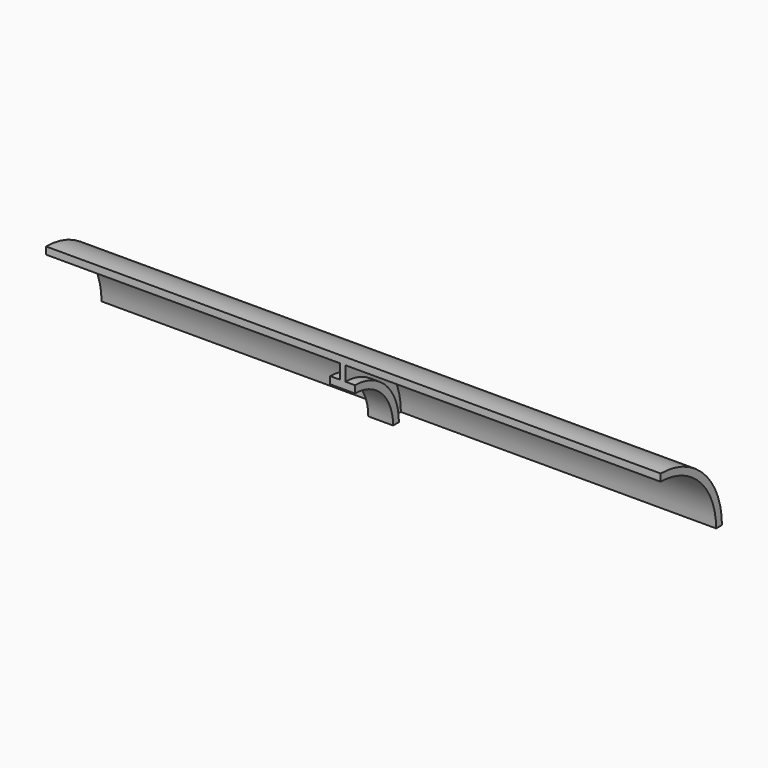
from build123d import *

# Parameters (mm, degrees)
F4_DEPTH = 1877.2339820862
F5_DEPTH = 1745.1422214508


# Not quite as in the source:
# - a feature of the source that left no trace in its solid (it failed there, or was rolled back) is left out


with BuildPart() as f2:
    # F2: sweep along a path in F1
    with BuildLine(Plane.YZ) as f2_path:
        ThreePointArc((0, 0), (269.4076836321, -111.5923163679), (381, -381))
    # F0 (on Front) → F2 (sweep)
    with BuildSketch(Plane.XZ):
        Polygon((76.2, 88.9), (0, 88.9), (-76.2, 88.9), (-76.2, 44.45), (-17.3748321831, 44.45), (-17.3748321831, 0), (-17.3748321831, -44.45), (-76.2, -44.45), (-76.2, -88.9), (0, -88.9), (76.2, -88.9), (76.2, -44.45), (17.3748321831, -44.45), (17.3748321831, 0), (17.3748321831, 44.45), (76.2, 44.45), align=None)
    sweep(path=f2_path.line)

    # F4 (add): a face of the model
    f4_faces = [f2.faces().sort_by_distance(p)[0] for p in [
        (76.2, 305.5375800558, -75.4624199442),
    ]]
    extrude(f4_faces, amount=F4_DEPTH)

    # F3 (on face) → F5 (join)
    with BuildSketch(Plane(origin=(-76.2, 0, 0), x_dir=(0, -1, 0), z_dir=(-1, 0, 0))):
        with BuildLine():
            Line((0, 44.45), (0, 88.9))
            ThreePointArc((0, 88.9), (-332.2694764796, -48.7305235204), (-469.9, -381))
            Line((-469.9, -381), (-425.45, -381))
            ThreePointArc((-425.45, -381), (-300.8385800558, -80.1614199442), (0, 44.45))
        make_face()
    extrude(amount=F5_DEPTH)


solid = f2.part
